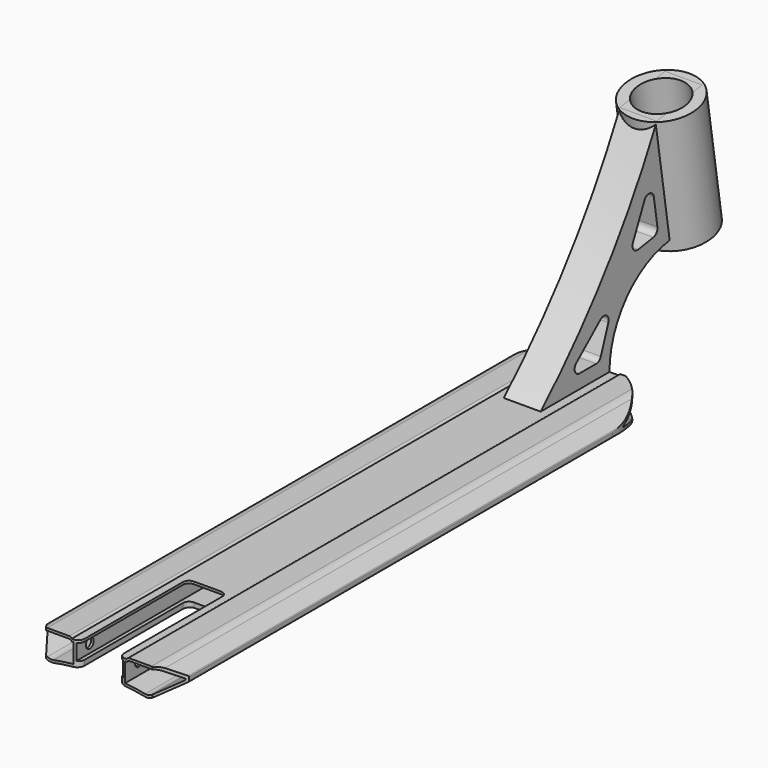
from build123d import *

# Parameters (mm, degrees)
F1_DEPTH       = 250
F2_W           = 38
F2_H           = 13
F3_DEPTH       = 250
F4_T1_DEPTH    = 509.3674969976
F5_R           = 9
F6_R           = 1
F7_W           = 38
F7_H           = 13
F8_DEPTH       = 500.001
F10_DEPTH      = 10.1555958277
F10_DEPTH_BACK = 13.3647093536
F12_DEPTH      = 10.1555959404
F12_DEPTH_BACK = 13.3647094536
F13_R          = 4.99999
F15_DEPTH      = 15
F16_R          = 29
F17_REACH      = 271.8612371718
F19_D          = 40
F21_D          = 8
F21_DEPTH      = 50
F21_TIP        = 2.4034424761
F23_DEPTH      = 72.5010001
F24_R          = 5


# Not quite as in the source:
# - a fillet or chamfer that OpenCascade refuses, or shapes differently, is made with other operations: its cross-section is extruded or revolved along the edge and cut away or added
# - a fillet or chamfer is up to 0.001 mm smaller than in the source, because OpenCascade refuses the exact size


with BuildPart() as f1:
    # F0 (on Front) → F1 (new body, symmetric)
    with BuildSketch(Plane.XZ):
        with BuildLine():
            Line((45.5824640741, 13.3637093536), (22.5, 13.3637093536))
            Line((22.5, 13.3637093536), (22.5, 12.0637093536))
            Line((22.5, 12.0637093536), (-22.5, 12.0637093536))
            Line((-22.5, 12.0637093536), (-22.5, 13.3637093536))
            Line((-22.5, 13.3637093536), (-45.5824640741, 13.3637093536))
            Line((-45.5824640741, 13.3637093536), (-57.5, 3.3637093536))
            Line((-57.5, 3.3637093536), (-57.5, -0.6362906464))
            Line((-57.5, -0.6362906464), (-40.1794919243, -10.6362906464))
            ThreePointArc((-40.1794919243, -10.6362906464), (0, -6.558745788), (40.1794919243, -10.6362906464))
            Line((40.1794919243, -10.6362906464), (57.5, -0.6362906464))
            Line((57.5, -0.6362906464), (57.5, 3.3637093536))
            Line((57.5, 3.3637093536), (45.5824640741, 13.3637093536))
        make_face()
    extrude(amount=F1_DEPTH, both=True)

    # F2 (on Front) → F3 (cut, symmetric)
    with BuildSketch(Plane.XZ):
        with Locations((0, 3.5637093536)):
            Rectangle(F2_W, F2_H)
    extrude(amount=F3_DEPTH, both=True, mode=Mode.SUBTRACT)

    # F4: fillet of radius 2 on 2 edges, made by hand

    # F4_s2 → F4_t1 (cut)
    with BuildSketch(Plane.XZ.offset(-254.6837484988)):
        with BuildLine():
            ThreePointArc((24.3734993995, 13.3637093536), (23.2333239744, 13.0068770261), (22.5, 12.0637093536))
            Line((22.5, 12.0637093536), (22.5, 13.3637093536))
            Line((22.5, 13.3637093536), (24.3734993995, 13.3637093536))
        make_face()
        with BuildLine():
            ThreePointArc((-22.5, 12.0637093536), (-23.2333239744, 13.0068770261), (-24.3734993995, 13.3637093536))
            Line((-24.3734993995, 13.3637093536), (-22.5, 13.3637093536))
            Line((-22.5, 13.3637093536), (-22.5, 12.0637093536))
        make_face()
    extrude(amount=F4_T1_DEPTH, mode=Mode.SUBTRACT)

    # F5
    f5_edges = [f1.edges().sort_by_distance(p)[0] for p in [
        (-45.582464, 0, 13.363709),
        (-40.179492, 0, -10.636291),
        (40.179492, 0, -10.636291),
        (45.582464, 0, 13.363709),
    ]]
    fillet(f5_edges, radius=F5_R)

    # F6
    f6_edges = [f1.edges().sort_by_distance(p)[0] for p in [
        (57.5, 0, 3.363709),
        (57.5, 0, -0.636291),
        (-57.5, 0, -0.636291),
        (-57.5, 0, 3.363709),
    ]]
    fillet(f6_edges, radius=F6_R)

    # F7 (on face) → F8 (cut, through all)
    with BuildSketch(Plane.XZ.offset(250)):
        with Locations((0, 3.5637093536)):
            Rectangle(F7_W, F7_H)
        with BuildLine():
            ThreePointArc((-42.1022690923, -7.2167736542), (-39.7790673433, -8.0549687072), (-37.3093701274, -8.0341606589))
            ThreePointArc((-37.3093701274, -8.0341606589), (-29.1789785809, -6.677312911), (-21, -5.6532953891))
            Line((-21, -5.6532953891), (-21, 10.0637093536))
            Line((-21, 10.0637093536), (-22.5, 10.0637093536))
            ThreePointArc((-22.5, 10.0637093536), (-23.2333239744, 11.0068770261), (-24.3734993995, 11.3637093536))
            Line((-24.3734993995, 11.3637093536), (-42.3067319657, 11.3637093536))
            ThreePointArc((-42.3067319657, 11.3637093536), (-44.7008729689, 10.9415576991), (-46.8062452335, 9.7260204554))
            Line((-46.8062452335, 9.7260204554), (-55.8572123903, 2.1313572523))
            ThreePointArc((-55.8572123903, 2.1313572523), (-56.109689349, 1.3031947048), (-55.6211874075, 0.5883774743))
            Line((-55.6211874075, 0.5883774743), (-42.1022690923, -7.2167736542))
        make_face()
        with BuildLine():
            Line((21, 10.0637093536), (21, -5.6532953891))
            ThreePointArc((21, -5.6532953891), (29.1789785809, -6.677312911), (37.3093701274, -8.0341606589))
            ThreePointArc((37.3093701274, -8.0341606589), (39.7790673433, -8.0549687072), (42.1022690923, -7.2167736542))
            Line((42.1022690923, -7.2167736542), (55.6211874075, 0.5883774743))
            ThreePointArc((55.6211874075, 0.5883774743), (56.109689349, 1.3031947048), (55.8572123903, 2.1313572523))
            Line((55.8572123903, 2.1313572523), (46.8062452335, 9.7260204554))
            ThreePointArc((46.8062452335, 9.7260204554), (44.7008729689, 10.9415576991), (42.3067319657, 11.3637093536))
            Line((42.3067319657, 11.3637093536), (24.3734993995, 11.3637093536))
            ThreePointArc((24.3734993995, 11.3637093536), (23.2333239744, 11.0068770261), (22.5, 10.0637093536))
            Line((22.5, 10.0637093536), (21, 10.0637093536))
        make_face()
    extrude(amount=-F8_DEPTH, mode=Mode.SUBTRACT)

    # F9 (on Top) → F10 (cut, two sides)
    with BuildSketch(Plane.XY) as f10_sk:
        with BuildLine():
            ThreePointArc((-57.5, 200), (0, 257.5), (57.5, 200))
            Line((57.5, 200), (57.5, 280))
            Line((57.5, 280), (-57.5, 280))
            Line((-57.5, 280), (-57.5, 200))
        make_face()
    extrude(amount=-F10_DEPTH, mode=Mode.SUBTRACT)
    extrude(f10_sk.sketch, amount=F10_DEPTH_BACK, mode=Mode.SUBTRACT)

    # F11 (on Top) → F12 (cut, two sides)
    with BuildSketch(Plane.XY) as f12_sk:
        Polygon((16, -140), (-16, -140), (-16, -250), (-43.2975540478, -250), (-68, -216), (-68, -346), (68, -346), (68, -216), (43.2975540478, -250), (16, -250), align=None)
    extrude(amount=-F12_DEPTH, mode=Mode.SUBTRACT)
    extrude(f12_sk.sketch, amount=F12_DEPTH_BACK, mode=Mode.SUBTRACT)

    # F13 (radius 5 in the source; OpenCascade refuses exactly that, so slightly less here)
    f13_edges = [f1.edges().sort_by_distance(p)[0] for p in [
        (16, -250, -5.068032),
        (-16, -250, -5.068032),
        (-16, -140, 11.063709),
        (16, -140, 11.063709),
        (-16, -140, -5.068032),
        (16, -140, -5.068032),
    ]]
    fillet(f13_edges, radius=F13_R)

    # F14 (on Right) → F15 (join, symmetric)
    with BuildSketch(Plane.YZ):
        with BuildLine():
            ThreePointArc((298.1274143767, 172.0339803398), (246.3607286322, 86.6508307745), (180.0101625919, 12.0339803398))
            Line((180.0101625919, 12.0339803398), (250.0101625919, 12.0339803398))
            ThreePointArc((250.0101625919, 12.0339803398), (268.6384602638, 59.5834093575), (314.6086825894, 81.8252692932))
            Line((314.6086825894, 81.8252692932), (316.0496527237, 73.6531215682))
            Line((316.0496527237, 73.6531215682), (361.3508093623, 81.6409377409))
            Line((361.3508093623, 81.6409377409), (344.1274143767, 179.3196645947))
            Line((344.1274143767, 179.3196645947), (298.1274143767, 172.0339803398))
        make_face()
    extrude(amount=F15_DEPTH, both=True)

    f17_end = Plane(origin=(0, 338.700231043, 77.6470296545), x_dir=(0, -0.984807753, -0.1736481777), z_dir=(0, 0.1736481777, -0.984807753))
    # F16 (on face) → F17 (join, up to a plane its end follows)
    with BuildSketch(Plane(origin=(0, -19.2850146437, 121.7607904173), x_dir=(1, 0, 0), z_dir=(0, -0.156434465, 0.9876883406))):
        with Locations((0, 344.9424106611)):
            Circle(F16_R)
    f17_long = extrude(amount=-F17_REACH, mode=Mode.PRIVATE)
    add(split(f17_long, bisect_by=f17_end, keep=Keep.BOTTOM, mode=Mode.PRIVATE))

    # F19 (through all)
    with Locations(Plane(origin=(0, -19.2850146437, 121.7607904173), x_dir=(1, 0, 0), z_dir=(0, -0.156434465, 0.9876883406))):
        with Locations((0, 344.9424106611)):
            Hole(F19_D / 2)

    # F21 (one way)
    with BuildSketch(Plane.YZ.offset(21)):
        with Locations((-236, 4.3467046109)):
            Circle(F21_D / 2)
    extrude(amount=-F21_DEPTH, mode=Mode.SUBTRACT)
    with Locations(Plane.YZ.offset(21)):
        with Locations((-236, 4.3467046109)):
            with Locations((0, 0, -(F21_DEPTH + F21_TIP / 2))):  # 118° drill point
                Cone(0, F21_D / 2, F21_TIP, mode=Mode.SUBTRACT)

    # F22 (on face) → F23 (cut, through all)
    with BuildSketch(Plane.YZ.offset(15)):
        Polygon((299.5670397655, 91.0553244288), (292.5274888387, 135.5012997556), (269.9363895476, 86.3622904776), align=None)
        Polygon((240, 23.3637093536), (255.3909064497, 65.6498772889), (206, 23.3637093536), align=None)
    extrude(amount=-F23_DEPTH, mode=Mode.SUBTRACT)

    # F24
    f24_edges = [f1.edges().sort_by_distance(p)[0] for p in [
        (0, 269.93639, 86.36229),
        (0, 292.527489, 135.5013),
        (0, 299.56704, 91.055324),
        (0, 206, 23.363709),
        (0, 255.390906, 65.649877),
        (0, 240, 23.363709),
    ]]
    fillet(f24_edges, radius=F24_R)


solid = f1.part
